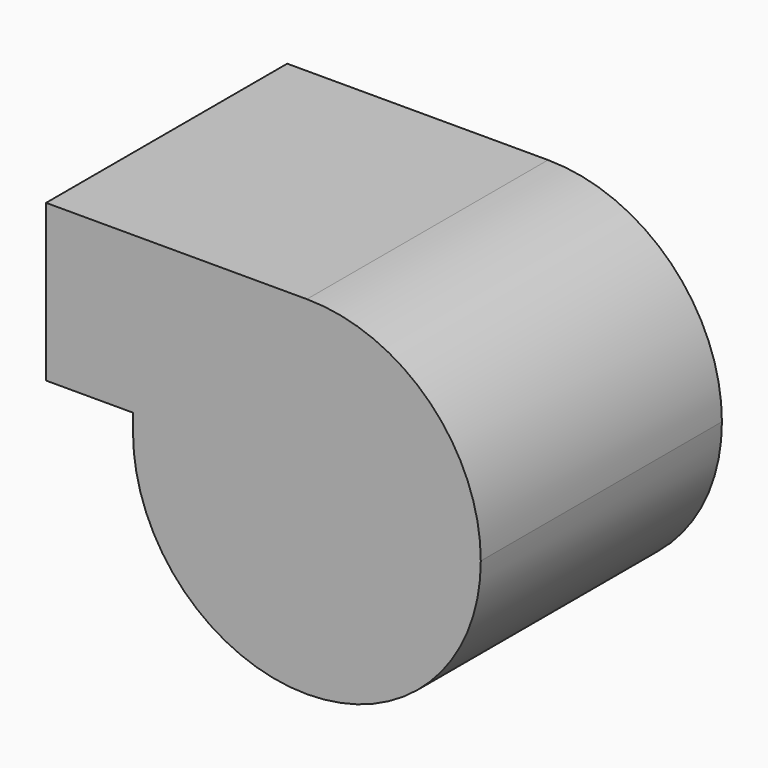
from build123d import *

# Parameters (mm, degrees)
F0_W     = 600
F0_H     = 600
F1_DEPTH = 520
F2_R     = 299.99999
F3_W     = 520
F3_H     = 270
F3_W_2   = 500
F3_H_2   = 250
F4_DEPTH = 150
F5_R     = 25
F6_DEPTH = 300


# Not quite as in the source:
# - a fillet or chamfer is up to 0.001 mm smaller than in the source, because OpenCascade refuses the exact size


with BuildPart() as f1:
    # F0 (on Front) → F1 (new body)
    with BuildSketch(Plane.XZ):
        Rectangle(F0_W, F0_H)
    extrude(amount=F1_DEPTH)

    # F2 (radius 300 in the source; OpenCascade refuses exactly that, so slightly less here)
    f2_edges = [f1.edges().sort_by_distance(p)[0] for p in [
        (300, -260, 300),
        (300, -260, -300),
        (-300, -260, -300),
    ]]
    fillet(f2_edges, radius=F2_R)

    # F3 (on face) → F4 (join)
    with BuildSketch(Plane(origin=(-300, 0, 0), x_dir=(0, -1, 0), z_dir=(-1, 0, 0))):
        with Locations((260, 165)):
            Rectangle(F3_W, F3_H)
        with Locations((260, 165)):
            Rectangle(F3_W_2, F3_H_2, mode=Mode.SUBTRACT)
    extrude(amount=F4_DEPTH)

    # F5 (on face) → F6 (cut)
    with BuildSketch(Plane(origin=(0, 0, 0), x_dir=(-1, 0, 0), z_dir=(0, 1, 0))):
        Circle(F5_R)
    extrude(amount=-F6_DEPTH, mode=Mode.SUBTRACT)


solid = f1.part
